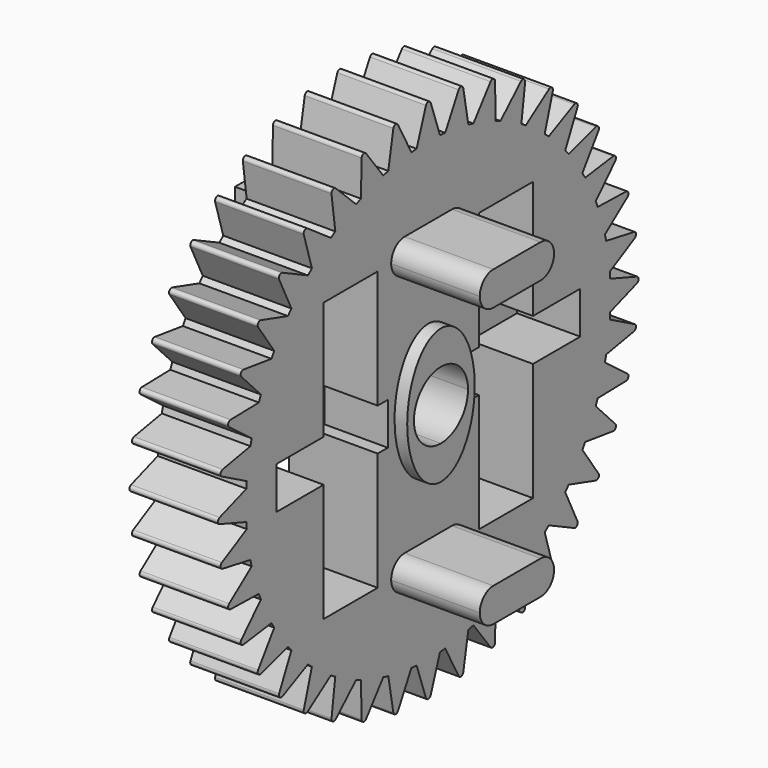
from build123d import *

# Parameters (mm, degrees)
F0_R          = 13.716
F1_DEPTH      = 5.334
F2_DEPTH      = 6.096
F2_DEPTH_BACK = 1.016
F3_DEPTH      = 1.524
F4_DEPTH      = 10.668
F4_DEPTH_BACK = 4.064
F5_R          = 1.01599
F7_DEPTH      = 5.334
F8_R          = 0.187954292
F9_COUNT      = 40


# Not quite as in the source:
# - a fillet or chamfer is up to 0.001 mm smaller than in the source, because OpenCascade refuses the exact size


with BuildPart() as f1:
    # F0 (on Right) → F1 (new body)
    with BuildSketch(Plane.YZ):
        Circle(F0_R)
        Polygon((2.794, -7.366), (2.794, -8.382), (2.794, -9.398), (-2.794, -9.398), (-2.794, -8.382), (-2.794, -7.366), align=None, mode=Mode.SUBTRACT)
        Polygon((-3.81, 8.382), (-3.81, 1.27), (-3.048, 1.27), (-3.048, 0), (-3.048, -1.27), (-3.81, -1.27), (-3.81, -8.382), (-7.874, -8.382), (-7.874, -1.27), (-11.43, -1.27), (-11.43, 0), (-11.43, 1.27), (-7.874, 1.27), (-7.874, 8.382), align=None, mode=Mode.SUBTRACT)
        with BuildLine():
            add(Edge.make_bspline(
                [(0, 4.064), (-2.54, 4.064), (-2.54, 0)],
                knots=[0, 0, 0, 1.5707963268, 1.5707963268, 1.5707963268], degree=2, weights=[1, 0.7071067812, 1]))
            add(Edge.make_bspline(
                [(2.54, 0), (2.54, 4.064), (0, 4.064)],
                knots=[4.7123889804, 4.7123889804, 4.7123889804, 6.2831853072, 6.2831853072, 6.2831853072], degree=2, weights=[1, 0.7071067812, 1]))
            add(Edge.make_bspline(
                [(0, -4.064), (2.54, -4.064), (2.54, 0)],
                knots=[3.1415926536, 3.1415926536, 3.1415926536, 4.7123889804, 4.7123889804, 4.7123889804], degree=2, weights=[1, 0.7071067812, 1]))
            add(Edge.make_bspline(
                [(-2.54, 0), (-2.54, -4.064), (0, -4.064)],
                knots=[1.5707963268, 1.5707963268, 1.5707963268, 3.1415926536, 3.1415926536, 3.1415926536], degree=2, weights=[1, 0.7071067812, 1]))
        make_face(mode=Mode.SUBTRACT)
        Polygon((3.048, 1.27), (3.81, 1.27), (3.81, 8.382), (7.874, 8.382), (7.874, 1.27), (11.43, 1.27), (11.43, 0), (11.43, -1.27), (7.874, -1.27), (7.874, -8.382), (3.81, -8.382), (3.81, -1.27), (3.048, -1.27), (3.048, 0), align=None, mode=Mode.SUBTRACT)
        Polygon((-2.794, 7.366), (-2.794, 8.382), (-2.794, 9.398), (2.794, 9.398), (2.794, 8.382), (2.794, 7.366), align=None, mode=Mode.SUBTRACT)
    extrude(amount=F1_DEPTH)

    # F0 (on Right) → F2 (join, two sides)
    with BuildSketch(Plane.YZ) as f2_sk:
        with BuildLine():
            ThreePointArc((-2.032, 0), (-1.4368409794, 1.4368409794), (0, 2.032))
            Line((0, 2.032), (0, 4.064))
            add(Edge.make_bspline(
                [(0, 4.064), (-2.54, 4.064), (-2.54, 0)],
                knots=[0, 0, 0, 1.5707963268, 1.5707963268, 1.5707963268], degree=2, weights=[1, 0.7071067812, 1]))
            Line((-2.54, 0), (-2.032, 0))
        make_face()
        with BuildLine():
            Line((0, 4.064), (0, 2.032))
            ThreePointArc((0, 2.032), (1.4368409794, 1.4368409794), (2.032, 0))
            Line((2.032, 0), (2.54, 0))
            add(Edge.make_bspline(
                [(2.54, 0), (2.54, 4.064), (0, 4.064)],
                knots=[4.7123889804, 4.7123889804, 4.7123889804, 6.2831853072, 6.2831853072, 6.2831853072], degree=2, weights=[1, 0.7071067812, 1]))
        make_face()
        with BuildLine():
            ThreePointArc((2.032, 0), (1.4368409794, -1.4368409794), (0, -2.032))
            Line((0, -2.032), (0, -4.064))
            add(Edge.make_bspline(
                [(0, -4.064), (2.54, -4.064), (2.54, 0)],
                knots=[3.1415926536, 3.1415926536, 3.1415926536, 4.7123889804, 4.7123889804, 4.7123889804], degree=2, weights=[1, 0.7071067812, 1]))
            Line((2.54, 0), (2.032, 0))
        make_face()
        with BuildLine():
            Line((0, -4.064), (0, -2.032))
            ThreePointArc((0, -2.032), (-1.4368409794, -1.4368409794), (-2.032, 0))
            Line((-2.032, 0), (-2.54, 0))
            add(Edge.make_bspline(
                [(-2.54, 0), (-2.54, -4.064), (0, -4.064)],
                knots=[1.5707963268, 1.5707963268, 1.5707963268, 3.1415926536, 3.1415926536, 3.1415926536], degree=2, weights=[1, 0.7071067812, 1]))
        make_face()
    extrude(amount=F2_DEPTH)
    extrude(f2_sk.sketch, amount=-F2_DEPTH_BACK)

    # F0 (on Right) → F3 (join)
    with BuildSketch(Plane.YZ):
        Polygon((-7.874, -1.27), (-7.874, 1.27), (-11.43, 1.27), (-11.43, 0), (-11.43, -1.27), align=None)
        Polygon((11.43, 1.27), (7.874, 1.27), (7.874, -1.27), (11.43, -1.27), (11.43, 0), align=None)
        Polygon((-3.81, 1.27), (-3.81, 0), (-3.81, -1.27), (-3.048, -1.27), (-3.048, 0), (-3.048, 1.27), align=None)
        Polygon((3.81, -1.27), (3.81, 0), (3.81, 1.27), (3.048, 1.27), (3.048, 0), (3.048, -1.27), align=None)
    extrude(amount=F3_DEPTH)

    # F0 (on Right) → F4 (join, two sides)
    with BuildSketch(Plane.YZ) as f4_sk:
        Polygon((-2.794, 8.382), (0, 8.382), (2.794, 8.382), (2.794, 9.398), (-2.794, 9.398), align=None)
        Polygon((2.794, -8.382), (0, -8.382), (-2.794, -8.382), (-2.794, -9.398), (2.794, -9.398), align=None)
        Polygon((-2.794, -8.382), (0, -8.382), (2.794, -8.382), (2.794, -7.366), (-2.794, -7.366), align=None)
        Polygon((2.794, 8.382), (0, 8.382), (-2.794, 8.382), (-2.794, 7.366), (2.794, 7.366), align=None)
    extrude(amount=F4_DEPTH)
    extrude(f4_sk.sketch, amount=-F4_DEPTH_BACK)

    # F5 (radius 1.016 in the source; OpenCascade refuses exactly that, so slightly less here)
    f5_edges = [f1.edges().sort_by_distance(p)[0] for p in [
        (8.001, 2.794, 9.398),
        (8.001, 2.794, 7.366),
        (8.001, -2.794, 9.398),
        (8.001, -2.794, 7.366),
        (8.001, -2.794, -7.366),
        (8.001, 2.794, -9.398),
        (8.001, 2.794, -7.366),
        (8.001, -2.794, -9.398),
    ]]
    fillet(f5_edges, radius=F5_R)



with BuildPart() as f7:
    # F6 (on Right) → F7 (new body)
    with BuildSketch(Plane.YZ):
        Polygon((0, 16.2041655117), (-0.889, 13.6641655117), (0, 13.6641655117), align=None)
        Polygon((0, 16.2041655117), (0, 13.6641655117), (0.889, 13.6641655117), align=None)
    extrude(amount=F7_DEPTH)

    # F8
    f8_edges = [f7.edges().sort_by_distance(p)[0] for p in [
        (2.667, 0, 16.204166),
    ]]
    fillet(f8_edges, radius=F8_R)


with BuildPart() as f1_1:
    add(f1.part)

    add(f7.part)  # F9 merges F7
    # F9: F7 ×40 about axis
    f9_axis = Axis((5.334, 0, 0), (1, 0, 0))
    for i in range(1, F9_COUNT):
        add(f7.part.rotate(f9_axis, i * 360 / F9_COUNT))


solid = f1_1.part
